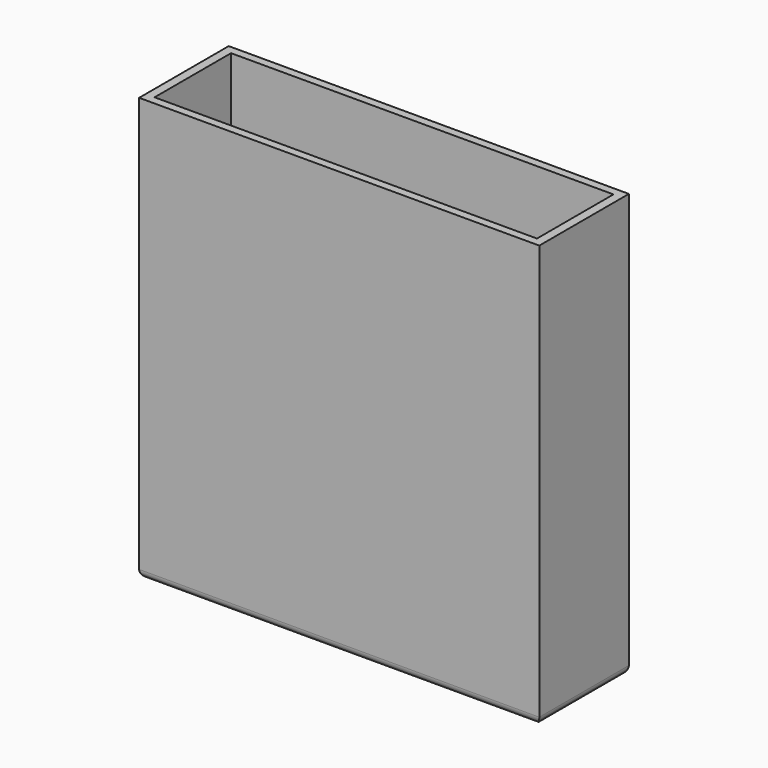
from build123d import *

# Parameters (mm, degrees)
F0_W     = 37.211
F0_H     = 39.37
F1_DEPTH = 5.207
F2_W     = 35.56
F2_H     = 8.89
F3_DEPTH = 39.37
F4_R     = 0.76199


# Not quite as in the source:
# - a fillet or chamfer is up to 0.001 mm smaller than in the source, because OpenCascade refuses the exact size


with BuildPart() as f1:
    # F0 (on Front) → F1 (new body, symmetric)
    with BuildSketch(Plane.XZ):
        Rectangle(F0_W, F0_H)
    extrude(amount=F1_DEPTH, both=True)

    # F2 (on face) → F3 (cut)
    with BuildSketch(Plane.XY.offset(19.685)):
        Rectangle(F2_W, F2_H)
    extrude(amount=-F3_DEPTH, mode=Mode.SUBTRACT)

    # F4 (radius 0.762 in the source; OpenCascade refuses exactly that, so slightly less here)
    f4_edges = [f1.edges().sort_by_distance(p)[0] for p in [
        (18.6055, 0, -19.685),
        (0, -5.207, -19.685),
        (0, 5.207, -19.685),
        (-18.6055, 0, -19.685),
    ]]
    fillet(f4_edges, radius=F4_R)


solid = f1.part
